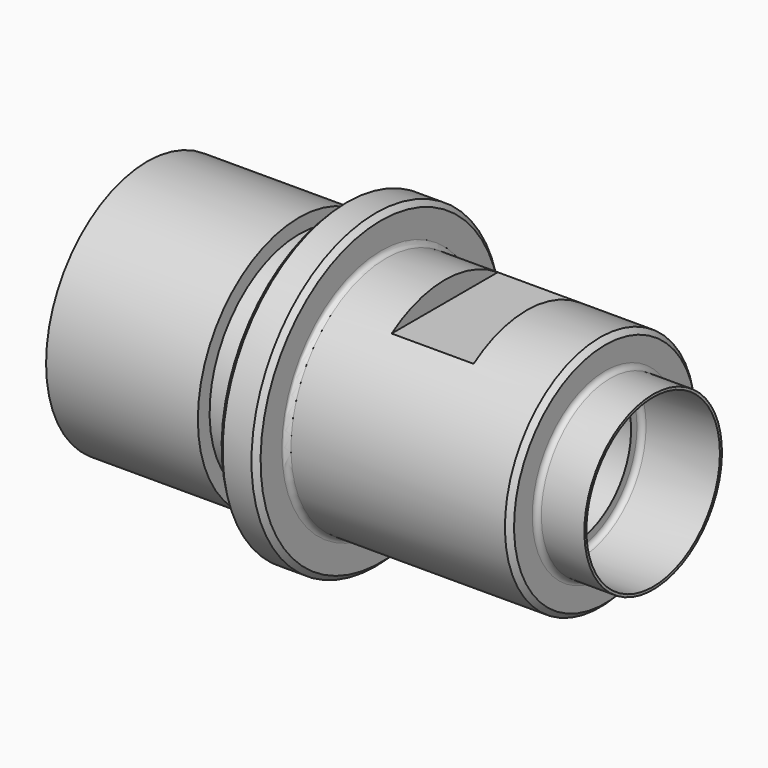
from build123d import *

# Parameters (mm, degrees)
F0_W           = 25.4
F0_H           = 2.7813
F2_W           = 1.9558
F2_H           = 1.4605
F4_W           = 13.6652
F4_H           = 2.921
F6_W           = 2.159
F6_H           = 3.2766
F6_W_2         = 2.413
F6_H_2         = 4.572
F8_R           = 3.6576
F9_DEPTH       = 10.541
F10_R          = 4.191
F11_DEPTH      = 3.9624
F12_W          = 4.1148
F12_H          = 3.937
F13_DEPTH      = 7.8115
F13_DEPTH_BACK = 7.8115
F14_SIZE       = 0.254
F15_SIZE       = 0.254
F16_R          = 0.254


# Not quite as in the source:
# - a feature of the source that left no trace in its solid (it failed there, or was rolled back) is left out


with BuildPart() as f1:
    # F0 (on Front) → F1 (revolve)
    with BuildSketch(Plane.XZ):
        with Locations((12.7, 4.95935)):
            Rectangle(F0_W, F0_H)
    revolve(axis=Axis((6.9021734883, 0, 0), (1, 0, 0)))

    # F2 (on Front) → F3 (revolve)
    with BuildSketch(Plane.XZ):
        with Locations((10.7569, 7.08025)):
            Rectangle(F2_W, F2_H)
    revolve(axis=Axis((12.3426117934, 0, 0), (1, 0, 0)))

    # F4 (on Front) → F5 (revolve, cut)
    with BuildSketch(Plane.XZ):
        with Locations((18.5674, 7.4295)):
            Rectangle(F4_W, F4_H)
    revolve(axis=Axis((16.2136404502, 0, 0), (1, 0, 0)), mode=Mode.SUBTRACT)

    # F6 (on Front) → F7 (revolve, cut)
    with BuildSketch(Plane.XZ):
        with Locations((8.6995, 7.2517)):
            Rectangle(F6_W, F6_H)
        with Locations((24.1935, 6.604)):
            Rectangle(F6_W_2, F6_H_2)
    revolve(axis=Axis((7.4812129023, 0, 0), (1, 0, 0)), mode=Mode.SUBTRACT)

    # F8 (on face) → F9 (cut)
    with BuildSketch(Plane(origin=(0, 0, 0), x_dir=(0, -1, 0), z_dir=(-1, 0, 0))):
        Circle(F8_R)
    extrude(amount=-F9_DEPTH, mode=Mode.SUBTRACT)

    # F10 (on face) → F11 (cut)
    with BuildSketch(Plane.YZ.offset(25.4)):
        Circle(F10_R)
    extrude(amount=-F11_DEPTH, mode=Mode.SUBTRACT)

    # F12 (on Front) → F13 (cut, two sides)
    with BuildSketch(Plane.XZ) as f13_sk:
        with Locations((16.9926, 6.9215)):
            Rectangle(F12_W, F12_H)
        with Locations((16.9926, -6.9215)):
            Rectangle(F12_W, F12_H)
    extrude(amount=-F13_DEPTH, mode=Mode.SUBTRACT)
    extrude(f13_sk.sketch, amount=F13_DEPTH_BACK, mode=Mode.SUBTRACT)

    # F14
    f14_edges = [f1.edges().sort_by_distance(p)[0] for p in [
        (9.779, 0, -7.8105),
        (11.7348, 0, -7.8105),
    ]]
    chamfer(f14_edges, length=F14_SIZE)

    # F15
    f15_edges = [f1.edges().sort_by_distance(p)[0] for p in [
        (22.987, 0, -5.969),
    ]]
    chamfer(f15_edges, length=F15_SIZE)

    # F16
    f16_edges = [f1.edges().sort_by_distance(p)[0] for p in [
        (9.779, 0, -5.6134),
        (11.7348, 0, -5.969),
        (22.987, 0, -4.318),
        (21.4376, -4.191, 0),
    ]]
    fillet(f16_edges, radius=F16_R)


solid = f1.part
